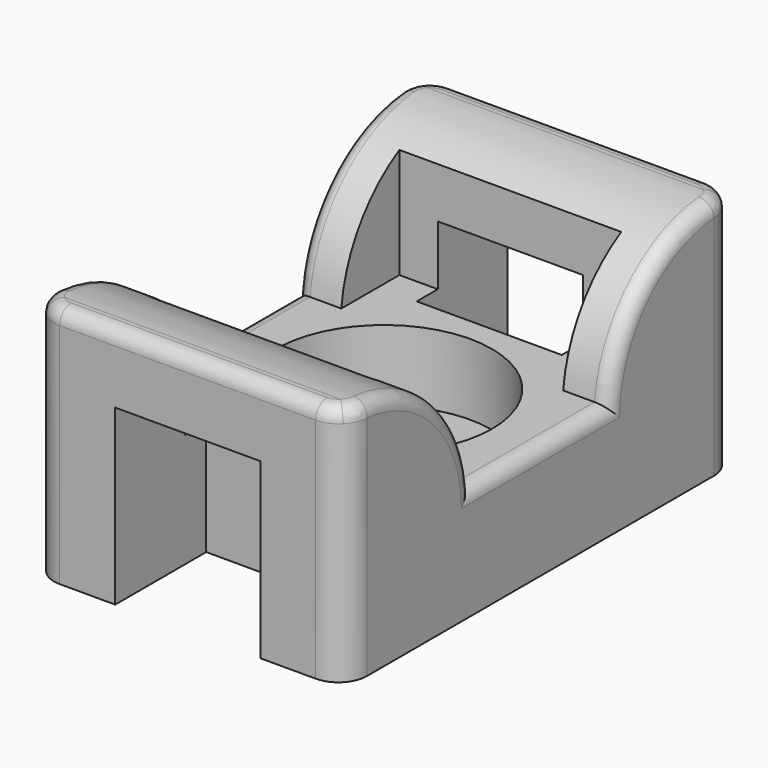
from build123d import *

# Parameters (mm, degrees)
F0_W         = 11
F0_H         = 17.25
F1_DEPTH     = 8.5
F2_W         = 7.8
F2_H         = 2.55
F2_H_2       = 6
F2_W_2       = 1.6
F3_DEPTH     = 4.5
F4_W         = 5.1
F4_H         = 4
F5_DEPTH     = 6.1
F6_R         = 3.8
F7_DEPTH     = 2.5
F8_R         = 1.9
F9_DEPTH     = 1.501
F10_T1_DEPTH = 26.4746859277
F11_R        = 1
F12_R        = 0.5


# Not quite as in the source:
# - a fillet or chamfer that OpenCascade refuses, or shapes differently, is made with other operations: its cross-section is extruded or revolved along the edge and cut away or added


with BuildPart() as f1:
    # F0 (on Top) → F1 (new body)
    with BuildSketch(Plane.XY):
        Rectangle(F0_W, F0_H)
    extrude(amount=F1_DEPTH)

    # F2 (on face) → F3 (cut)
    with BuildSketch(Plane.XY.offset(8.5)):
        with Locations((0, -4.275)):
            Rectangle(F2_W, F2_H)
        Rectangle(F2_W, F2_H_2)
        with Locations((4.7, 0)):
            Rectangle(F2_W_2, F2_H_2)
        with Locations((-4.7, 0)):
            Rectangle(F2_W_2, F2_H_2)
        with Locations((0, 4.275)):
            Rectangle(F2_W, F2_H)
    extrude(amount=-F3_DEPTH, mode=Mode.SUBTRACT)

    # F4 (on face) → F5 (cut)
    with BuildSketch(Plane(origin=(0, 0, 0), x_dir=(1, 0, 0), z_dir=(0, 0, -1))):
        with Locations((0, -6.625)):
            Rectangle(F4_W, F4_H)
        with Locations((0, 6.625)):
            Rectangle(F4_W, F4_H)
    extrude(amount=-F5_DEPTH, mode=Mode.SUBTRACT)

    # F6 (on face) → F7 (cut)
    with BuildSketch(Plane.XY.offset(4)):
        Circle(F6_R)
    extrude(amount=-F7_DEPTH, mode=Mode.SUBTRACT)

    # F8 (on face) → F9 (cut, through all)
    with BuildSketch(Plane.XY.offset(1.5)):
        Circle(F8_R)
    extrude(amount=-F9_DEPTH, mode=Mode.SUBTRACT)

    # F10: fillet of radius 5 on 2 edges, made by hand

    # F10_s2 → F10_t1 (cut)
    with BuildSketch(Plane.YZ.offset(-17.9373429638)):
        with BuildLine():
            ThreePointArc((-7.9749371855, 8.5), (-4.6208352193, 7.2080992435), (-3, 4))
            Line((-3, 4), (-3, 8.5))
            Line((-3, 8.5), (-7.9749371855, 8.5))
        make_face()
        with BuildLine():
            ThreePointArc((7.9749371855, 8.5), (4.6208352193, 7.2080992435), (3, 4))
            Line((3, 4), (3, 8.5))
            Line((3, 8.5), (7.9749371855, 8.5))
        make_face()
    extrude(amount=F10_T1_DEPTH, mode=Mode.SUBTRACT)

    # F11
    f11_edges = [f1.edges().sort_by_distance(p)[0] for p in [
        (5.5, -8.625, 4.25),
        (-5.5, -8.625, 4.25),
        (5.5, 8.625, 4.25),
        (-5.5, 8.625, 4.25),
    ]]
    fillet(f11_edges, radius=F11_R)

    # F12
    f12_edges = [f1.edges().sort_by_distance(p)[0] for p in [
        (0, 8.625, 8.5),
        (0, -8.625, 8.5),
        (-5.5, 0, 4),
        (5.5, 0, 4),
        (5.5, -4.493052, 7.088381),
        (5.5, 4.493052, 7.088381),
        (5.483858, -7.803952, 8.497076),
        (5.070115, -8.446565, 8.5),
        (5.483858, 7.803952, 8.497076),
        (5.070115, 8.446565, 8.5),
        (-5.5, -4.493052, 7.088381),
        (-5.483858, -7.803951, 8.497076),
        (-5.5, 4.493052, 7.088381),
        (-5.483858, 7.803952, 8.497076),
        (-5.070115, -8.446565, 8.5),
        (-5.070115, 8.446565, 8.5),
    ]]
    fillet(f12_edges, radius=F12_R)


solid = f1.part
